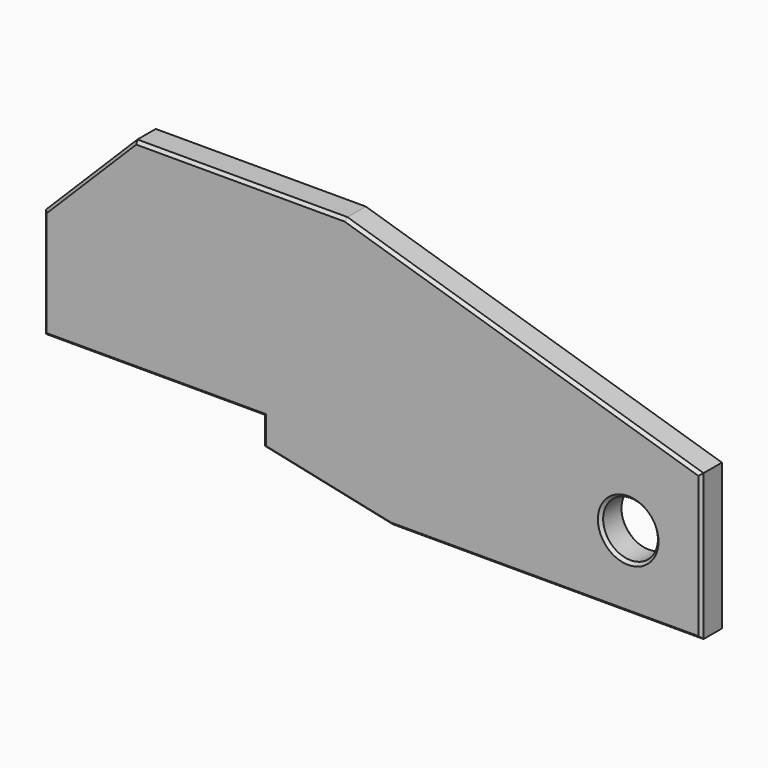
from build123d import *

# Parameters (mm, degrees)
F0_R     = 9.525
F1_DEPTH = 10
F2_SIZE  = 1.016


# Not quite as in the source:
# - a feature names something its author has since deleted; it is built from what else it names


with BuildPart() as f1:
    # F0 (on Front) → F1 (new body)
    with BuildSketch(Plane.XZ):
        Polygon((0, 38.1), (0, 0), (76.2, 0), (76.2, -9.525), (120.65, -19.05), (228.6, -19.05), (228.6, 31.75), (104.775, 69.85), (31.75, 69.85), align=None)
        with Locations((203.2, 6.35)):
            Circle(F0_R, mode=Mode.SUBTRACT)
    extrude(amount=F1_DEPTH)

    # F2
    f2_edges = [f1.edges().sort_by_distance(p)[0] for p in [
        (15.875, -10, 53.975),
        (0, -10, 19.05),
        (38.1, -10, 0),
        (76.2, -10, -4.7625),
        (98.425, -10, -14.2875),
        (174.625, -10, -19.05),
        (228.6, -10, 6.35),
        (166.6875, -10, 50.8),
        (68.2625, -10, 69.85),
        (193.675, -10, 6.35),
        (15.875, 0, 53.975),
        (0, 0, 19.05),
        (38.1, 0, 0),
        (76.2, 0, -4.7625),
        (98.425, 0, -14.2875),
        (174.625, 0, -19.05),
        (228.6, 0, 6.35),
        (166.6875, 0, 50.8),
        (68.2625, 0, 69.85),
        (193.675, 0, 6.35),
    ]]
    chamfer(f2_edges, length=F2_SIZE)


solid = f1.part
